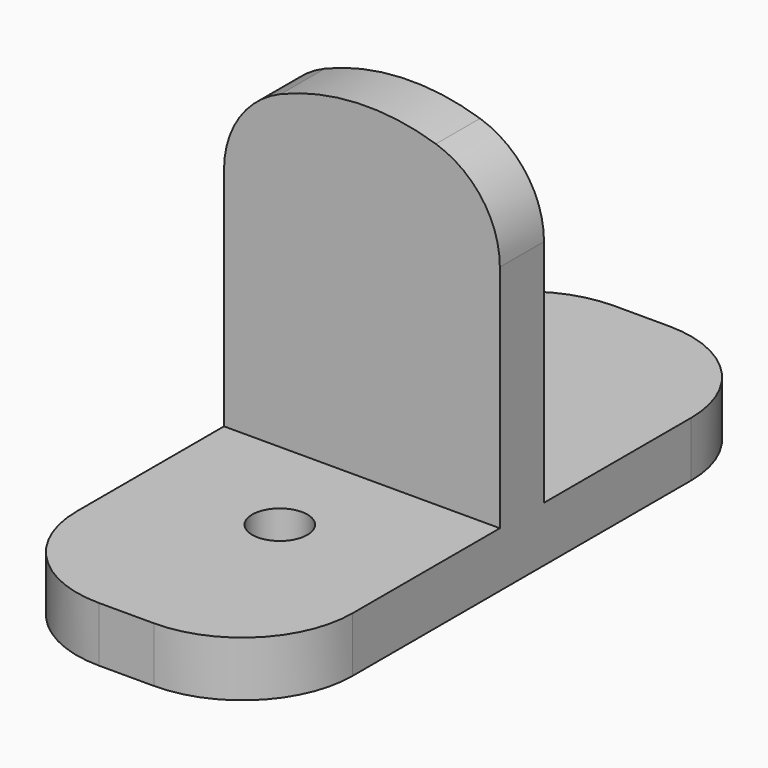
from build123d import *

# Parameters (mm, degrees)
F1_DEPTH = 3.81
F2_R     = 6.35
F3_W     = 19.05
F3_H     = 44.45
F4_DEPTH = 3.81
F5_R     = 7.62
F6_R     = 1.905
F6_R_2   = 1.9053216062
F7_DEPTH = 25.4


# Not quite as in the source:
# - a feature names something its author has since deleted; it is built from what else it names


with BuildPart() as f1:
    # F0 (on Front) → F1 (new body)
    with BuildSketch(Plane.XZ):
        with BuildLine():
            Line((0, 19.1190056503), (0, 0))
            Line((0, 0), (19.05, 0))
            Line((19.05, 0), (19.05, 19.6883492172))
            ThreePointArc((19.05, 19.6883492172), (9.4277487791, 22.6576630171), (0, 19.1190056503))
        make_face()
    extrude(amount=F1_DEPTH)

    # F2
    f2_edges = [f1.edges().sort_by_distance(p)[0] for p in [
        (0, -1.905, 19.119006),
        (19.05, -1.905, 19.688349),
    ]]
    fillet(f2_edges, radius=F2_R)

    # F3 (on face) → F4 (join)
    with BuildSketch(Plane(origin=(0, 0, 0), x_dir=(1, 0, 0), z_dir=(0, 0, -1))):
        with Locations((9.525, 1.905)):
            Rectangle(F3_W, F3_H)
    extrude(amount=F4_DEPTH)

    # F5
    f5_edges = [f1.edges().sort_by_distance(p)[0] for p in [
        (19.05, -24.13, -1.905),
        (0, -24.13, -1.905),
        (19.05, 20.32, -1.905),
        (0, 20.32, -1.905),
    ]]
    fillet(f5_edges, radius=F5_R)

    # F6 (on face) → F7 (cut)
    with BuildSketch(Plane.XY):
        with Locations((9.525, 7.3555377312)):
            Circle(F6_R)
        with Locations((9.525, -10.8990902081)):
            Circle(F6_R_2)
    extrude(amount=-F7_DEPTH, mode=Mode.SUBTRACT)


solid = f1.part
